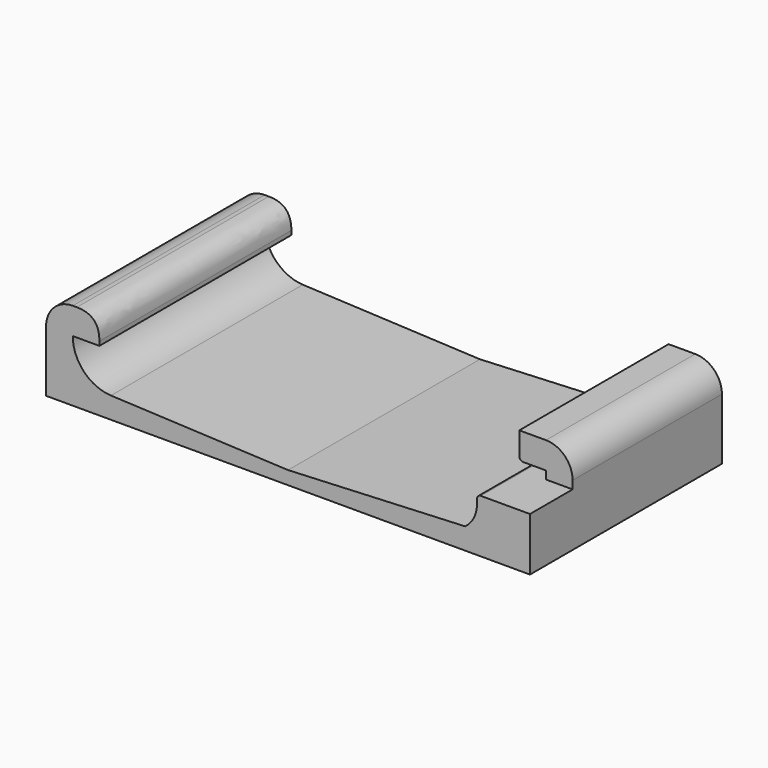
from build123d import *

# Parameters (mm, degrees)
F1_DEPTH    = 22.86
F2_R        = 5.08
F3_R        = 0.762
F4_R        = 0.762
F5_W        = 14.2031247761
F5_H        = 10.16
F6_DEPTH    = 6.604
F7_T1_DEPTH = 67.1823585695


# Not quite as in the source:
# - a fillet or chamfer that OpenCascade refuses, or shapes differently, is made with other operations: its cross-section is extruded or revolved along the edge and cut away or added


with BuildPart() as f1:
    # F0 (on Front) → F1 (new body, symmetric)
    with BuildSketch(Plane.XZ):
        with BuildLine():
            Line((-35.941, 20.9608385392), (-46.101, 20.9608385392))
            Line((-46.101, 20.9608385392), (-46.101, 4.1968385392))
            Line((-46.101, 4.1968385392), (0, 4.1968385392))
            Line((0, 4.1968385392), (46.101, 4.1968385392))
            Line((46.101, 4.1968385392), (46.101, 20.9608385392))
            Line((46.101, 20.9608385392), (35.941, 20.9608385392))
            Line((35.941, 20.9608385392), (35.941, 15.8808385392))
            Line((35.941, 15.8808385392), (41.021, 15.8808385392))
            Line((41.021, 15.8808385392), (41.021, 14.3568385392))
            Line((41.021, 14.3568385392), (35.9785540412, 14.3568385392))
            Line((35.9785540412, 14.3568385392), (36.0038614542, 12.846416393))
            ThreePointArc((36.0038614542, 12.846416393), (35.4291085131, 10.2844081543), (33.7465347616, 8.2686768405))
            Line((33.7465347616, 8.2686768405), (0, 6.7368385392))
            Line((0, 6.7368385392), (-33.7465347616, 8.2686768405))
            ThreePointArc((-33.7465347616, 8.2686768405), (-38.9099642803, 10.6162670887), (-41.021, 15.8808385392))
            Line((-41.021, 15.8808385392), (-35.941, 15.8808385392))
            Line((-35.941, 15.8808385392), (-35.941, 20.9608385392))
        make_face()
    extrude(amount=F1_DEPTH, both=True)

    # F2
    f2_edges = [f1.edges().sort_by_distance(p)[0] for p in [
        (-46.101, 0, 20.960839),
        (46.101, 0, 20.960839),
    ]]
    fillet(f2_edges, radius=F2_R)

    # F3
    f3_edges = [f1.edges().sort_by_distance(p)[0] for p in [
        (35.978554, 0, 14.356839),
    ]]
    fillet(f3_edges, radius=F3_R)

    # F4
    f4_edges = [f1.edges().sort_by_distance(p)[0] for p in [
        (35.941, 0, 15.880839),
    ]]
    fillet(f4_edges, radius=F4_R)

    # F5 (on face) → F6 (cut, through all)
    with BuildSketch(Plane.XY.offset(20.9608385392)):
        with Locations((43.0425623881, -17.78)):
            Rectangle(F5_W, F5_H)
    extrude(amount=-F6_DEPTH, mode=Mode.SUBTRACT)

    # F7: fillet of radius 4.2924717139 on 1 edges, made by hand

    # F7_s2 → F7_t1 (cut)
    with BuildSketch(Plane.XZ.offset(-33.5911792847)):
        with BuildLine():
            add(Edge.make_bspline(
                [(-35.941, 16.6683668253), (-35.941, 20.9608385392), (-40.2334717139, 20.9608385392)],
                knots=[0, 0, 0, 1, 1, 1], degree=2, weights=[1, 1, 1]))
            Line((-40.2334717139, 20.9608385392), (-35.941, 20.9608385392))
            Line((-35.941, 20.9608385392), (-35.941, 16.6683668253))
        make_face()
    extrude(amount=F7_T1_DEPTH, mode=Mode.SUBTRACT)


solid = f1.part
